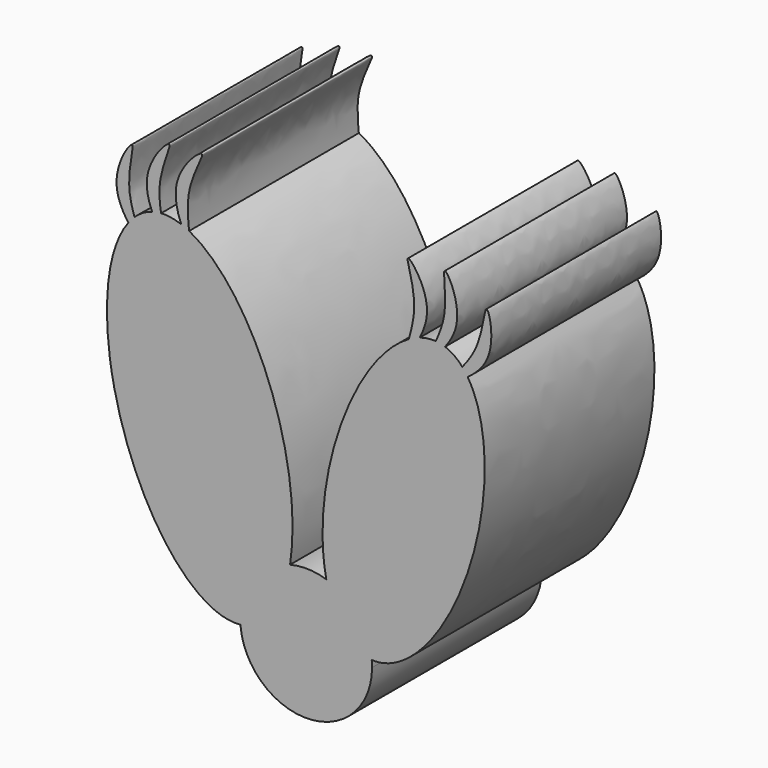
from build123d import *

# Parameters (mm, degrees)
F1_DEPTH = 25.4


# Not quite as in the source:
# - a feature of the source that left no trace in its solid (it failed there, or was rolled back) is left out


with BuildPart() as f1:
    # F0 (on Front) → F1 (new body)
    with BuildSketch(Plane.XZ):
        with BuildLine():
            ThreePointArc((-7.8657495184, -0.5963303534), (0.2983787071, -7.8826769263), (7.8883220888, 0))
            ThreePointArc((7.8883220888, 0), (7.8783514063, 0.396490223), (7.848464564, 0.7919781345))
            add(Edge.make_bspline(
                [(2.4115413859, 7.5106653182), (3.7514217892, 1.0542595546), (7.848464564, 0.7919781345)],
                knots=[2.3709530861, 2.3709530861, 2.3709530861, 3.2318966265, 3.2318966265, 3.2318966265], degree=2, weights=[1, 0.9087689813, 1]))
            ThreePointArc((2.4115413859, 7.5106653182), (0.2524493598, 7.8842814954), (-1.9261214081, 7.6495543464))
            add(Edge.make_bspline(
                [(-7.8657495184, -0.5963303534), (-3.1402244939, -0.0545859635), (-1.9261214081, 7.6495543464)],
                knots=[3.063961354, 3.063961354, 3.063961354, 3.9478311905, 3.9478311905, 3.9478311905], degree=2, weights=[1, 0.903925812, 1]))
        make_face()
        with BuildLine():
            add(Edge.make_bspline(
                [(2.4115413859, 7.5106653182), (3.7514217892, 1.0542595546), (7.848464564, 0.7919781345)],
                knots=[2.3709530861, 2.3709530861, 2.3709530861, 3.2318966265, 3.2318966265, 3.2318966265], degree=2, weights=[1, 0.9087689813, 1]))
            ThreePointArc((7.848464564, 0.7919781345), (6.1320567423, 4.9622077231), (2.4115413859, 7.5106653182))
        make_face()
        with BuildLine():
            ThreePointArc((2.4115413859, 7.5106653182), (6.1320567423, 4.9622077231), (7.848464564, 0.7919781345))
            add(Edge.make_bspline(
                [(7.848464564, 0.7919781345), (14.756882994, 0.3497201705), (19.3497784768, 13.7677159429), (23.9426739595, 27.1857117153), (19.3341341159, 34.3469906686)],
                knots=[3.2318966265, 3.2318966265, 3.2318966265, 4.5496269351, 4.5496269351, 5.8673572438, 5.8673572438, 5.8673572438], degree=2, weights=[1, 0.7906875156, 1, 0.7906875156, 1]))
            add(Edge.make_bspline(
                [(17.4727290869, 33.5254147649), (17.6220032936, 33.411960895), (18.4360560306, 33.7201138992), (19.3341341159, 34.3469906686)],
                knots=[0, 0, 0, 0, 0.1315254658, 0.1315254658, 0.1315254658, 0.1315254658], degree=3))
            add(Edge.make_bspline(
                [(18.6914906825, 35.2044384669), (17.9384272736, 34.2749423779), (17.3098526255, 33.649206847), (17.4727290869, 33.5254147649)],
                knots=[0.856489591, 0.856489591, 0.856489591, 0.856489591, 1, 1, 1, 1], degree=3))
            add(Edge.make_bspline(
                [(18.6914906825, 35.2044384669), (17.7756691464, 36.2476144498), (16.635683622, 36.651870342)],
                knots=[5.9688721424, 5.9688721424, 5.9688721424, 6.2406391942, 6.2406391942, 6.2406391942], degree=2, weights=[1, 0.9907820304, 1]))
            add(Edge.make_bspline(
                [(14.8701351136, 35.1549200714), (15.058499279, 35.0779113459), (15.8747352171, 35.6833048254), (16.635683622, 36.651870342)],
                knots=[0, 0, 0, 0, 0.1427509238, 0.1427509238, 0.1427509238, 0.1427509238], degree=3))
            add(Edge.make_bspline(
                [(15.5190667523, 36.8844184863), (15.0710606672, 35.9031366901), (14.6930112455, 35.2273334378), (14.8701351136, 35.1549200714)],
                knots=[0.8657674842, 0.8657674842, 0.8657674842, 0.8657674842, 1, 1, 1, 1], degree=3))
            add(Edge.make_bspline(
                [(15.5190667523, 36.8844184863), (14.5852576975, 36.9509876552), (13.5880398976, 36.6238878042)],
                knots=[0.0867629846, 0.0867629846, 0.0867629846, 0.2956399467, 0.2956399467, 0.2956399467], degree=2, weights=[1, 0.9945512572, 1]))
            add(Edge.make_bspline(
                [(12.1393091977, 34.898750484), (12.3347678279, 34.8563616726), (13.013036649, 35.5684327938), (13.5880398976, 36.6238878042)],
                knots=[0, 0, 0, 0, 0.14029874, 0.14029874, 0.14029874, 0.14029874], degree=3))
            add(Edge.make_bspline(
                [(12.2984461836, 36.0467759602), (12.1131626378, 35.3699550758), (11.9954319704, 34.9299529161), (12.1393091977, 34.898750484)],
                knots=[0.8967260045, 0.8967260045, 0.8967260045, 0.8967260045, 1, 1, 1, 1], degree=3))
            add(Edge.make_bspline(
                [(12.2984461836, 36.0467759602), (7.1738143092, 33.1518583115), (4.0152813166, 23.9954967618)],
                knots=[0.4297809871, 0.4297809871, 0.4297809871, 1.4031442636, 1.4031442636, 1.4031442636], degree=2, weights=[1, 0.8838897048, 1]))
            ThreePointArc((4.0152813166, 23.9954967618), (17.180368154, 14.7231281706), (2.1803673546, 8.8668232992))
            add(Edge.make_bspline(
                [(2.1803673546, 8.8668232992), (2.2756176481, 8.16563333), (2.4115413859, 7.5106653182)],
                knots=[2.2778551861, 2.2778551861, 2.2778551861, 2.3709530861, 2.3709530861, 2.3709530861], degree=2, weights=[1, 0.9989167932, 1]))
        make_face()
        with BuildLine():
            add(Edge.make_bspline(
                [(-16.8776699334, 5.1789570742), (-12.2994136592, -1.1046151815), (-7.8657495184, -0.5963303534)],
                knots=[2.2283826001, 2.2283826001, 2.2283826001, 3.063961354, 3.063961354, 3.063961354], degree=2, weights=[1, 0.9139881132, 1]))
            ThreePointArc((-7.8657495184, -0.5963303534), (-6.4006904066, 4.6105083989), (-1.9261214081, 7.6495543464))
            add(Edge.make_bspline(
                [(-1.9261214081, 7.6495543464), (1.7350735491, 30.881815249), (-14.0155701505, 38.8805496381)],
                knots=[3.9478311905, 3.9478311905, 3.9478311905, 5.8668053595, 5.8668053595, 5.8668053595], degree=2, weights=[1, 0.5739400867, 1]))
            add(Edge.make_bspline(
                [(-14.0155701505, 38.8805496381), (-13.9692331136, 38.3474513179), (-13.9585554591, 38.0149682113), (-14.0843456728, 38.01005632)],
                knots=[0.9116926893, 0.9116926893, 0.9116926893, 0.9116926893, 1, 1, 1, 1], degree=3))
            add(Edge.make_bspline(
                [(-14.0843456728, 38.01005632), (-14.2421212522, 38.0038954552), (-14.6145890314, 38.5130719057), (-14.9528763828, 39.2883132484)],
                knots=[0, 0, 0, 0, 0.1107616938, 0.1107616938, 0.1107616938, 0.1107616938], degree=3))
            add(Edge.make_bspline(
                [(-14.9528763828, 39.2883132484), (-16.2043765158, 39.7404083717), (-17.3655223204, 39.6654462324)],
                knots=[5.9522386597, 5.9522386597, 5.9522386597, 6.1810803974, 6.1810803974, 6.1810803974], degree=2, weights=[1, 0.9934610711, 1]))
            add(Edge.make_bspline(
                [(-17.3655223204, 39.6654462324), (-17.1795434662, 38.5086964495), (-16.9569761256, 37.6751636257), (-17.1571826672, 37.649743259)],
                knots=[0.8584303839, 0.8584303839, 0.8584303839, 0.8584303839, 1, 1, 1, 1], degree=3))
            add(Edge.make_bspline(
                [(-17.1571826672, 37.649743259), (-17.3543437255, 37.6247095794), (-17.9615142694, 38.3833898112), (-18.4409544135, 39.473830681)],
                knots=[0, 0, 0, 0, 0.1394161006, 0.1394161006, 0.1394161006, 0.1394161006], degree=3))
            add(Edge.make_bspline(
                [(-18.4409544135, 39.473830681), (-19.5878068307, 39.1314621905), (-20.5394386517, 38.2302190383)],
                knots=[0.0072900396, 0.0072900396, 0.0072900396, 0.2466181031, 0.2466181031, 0.2466181031], degree=2, weights=[1, 0.9928487993, 1]))
            add(Edge.make_bspline(
                [(-20.5394386517, 38.2302190383), (-20.1380049057, 37.0467661724), (-19.7331230605, 36.1979612039), (-19.9342295527, 36.1355692148)],
                knots=[0.8522933462, 0.8522933462, 0.8522933462, 0.8522933462, 1, 1, 1, 1], degree=3))
            add(Edge.make_bspline(
                [(-19.9342295527, 36.1355692148), (-20.102710459, 36.0832991028), (-20.6965090727, 36.5829791601), (-21.2904428927, 37.3886749603)],
                knots=[0, 0, 0, 0, 0.1237441449, 0.1237441449, 0.1237441449, 0.1237441449], degree=3))
            add(Edge.make_bspline(
                [(-21.2904428927, 37.3886749603), (-25.6133300033, 31.7080986333), (-22.9671125849, 19.4320361213)],
                knots=[0.3465956992, 0.3465956992, 0.3465956992, 1.4408599981, 1.4408599981, 1.4408599981], degree=2, weights=[1, 0.854020003, 1]))
            ThreePointArc((-22.9671125849, 19.4320361213), (-7.0630025292, 17.7995031872), (-16.8776699334, 5.1789570742))
        make_face()
        with BuildLine():
            ThreePointArc((-1.9261214081, 7.6495543464), (-6.4006904066, 4.6105083989), (-7.8657495184, -0.5963303534))
            add(Edge.make_bspline(
                [(-7.8657495184, -0.5963303534), (-3.1402244939, -0.0545859635), (-1.9261214081, 7.6495543464)],
                knots=[3.063961354, 3.063961354, 3.063961354, 3.9478311905, 3.9478311905, 3.9478311905], degree=2, weights=[1, 0.903925812, 1]))
        make_face()
        with BuildLine():
            add(Edge.make_bspline(
                [(17.4727290869, 33.5254147649), (17.6220032936, 33.411960895), (18.4360560306, 33.7201138992), (19.3341341159, 34.3469906686)],
                knots=[0, 0, 0, 0, 0.1315254658, 0.1315254658, 0.1315254658, 0.1315254658], degree=3))
            add(Edge.make_bspline(
                [(19.3341341159, 34.3469906686), (19.0317675739, 34.8168425581), (18.6914906825, 35.2044384669)],
                knots=[5.8673572438, 5.8673572438, 5.8673572438, 5.9688721424, 5.9688721424, 5.9688721424], degree=2, weights=[1, 0.9987121172, 1]))
            add(Edge.make_bspline(
                [(18.6914906825, 35.2044384669), (17.9384272736, 34.2749423779), (17.3098526255, 33.649206847), (17.4727290869, 33.5254147649)],
                knots=[0.856489591, 0.856489591, 0.856489591, 0.856489591, 1, 1, 1, 1], degree=3))
        make_face()
        with BuildLine():
            add(Edge.make_bspline(
                [(19.3341341159, 34.3469906686), (19.0317675739, 34.8168425581), (18.6914906825, 35.2044384669)],
                knots=[5.8673572438, 5.8673572438, 5.8673572438, 5.9688721424, 5.9688721424, 5.9688721424], degree=2, weights=[1, 0.9987121172, 1]))
            add(Edge.make_bspline(
                [(19.3341341159, 34.3469906686), (20.1798236278, 34.9372991482), (23.0009000721, 37.6134714521), (21.297221073, 45.0520380481), (21.2424649704, 38.6066952932), (19.2203684111, 35.8572251704), (18.6914906825, 35.2044384669)],
                knots=[0.1315254658, 0.1315254658, 0.1315254658, 0.1315254658, 0.2553785124, 0.5112252974, 0.7557019837, 0.856489591, 0.856489591, 0.856489591, 0.856489591], degree=3))
        make_face()
        with BuildLine():
            add(Edge.make_bspline(
                [(-22.9671125849, 19.4320361213), (-21.1623610737, 11.0596166006), (-16.8776699334, 5.1789570742)],
                knots=[1.4408599981, 1.4408599981, 1.4408599981, 2.2283826001, 2.2283826001, 2.2283826001], degree=2, weights=[1, 0.9234725177, 1]))
            ThreePointArc((-16.8776699334, 5.1789570742), (-7.0630025292, 17.7995031872), (-22.9671125849, 19.4320361213))
        make_face()
        with BuildLine():
            add(Edge.make_bspline(
                [(4.0152813166, 23.9954967618), (1.2243313225, 15.9047320704), (2.1803673546, 8.8668232992)],
                knots=[1.4031442636, 1.4031442636, 1.4031442636, 2.2778551861, 2.2778551861, 2.2778551861], degree=2, weights=[1, 0.9058749116, 1]))
            ThreePointArc((2.1803673546, 8.8668232992), (17.180368154, 14.7231281706), (4.0152813166, 23.9954967618))
        make_face()
        with BuildLine():
            add(Edge.make_bspline(
                [(-14.0155701505, 38.8805496381), (-13.9692331136, 38.3474513179), (-13.9585554591, 38.0149682113), (-14.0843456728, 38.01005632)],
                knots=[0.9116926893, 0.9116926893, 0.9116926893, 0.9116926893, 1, 1, 1, 1], degree=3))
            add(Edge.make_bspline(
                [(-14.0155701505, 38.8805496381), (-14.4874124644, 39.1201678667), (-14.9528763828, 39.2883132484)],
                knots=[5.8668053595, 5.8668053595, 5.8668053595, 5.9522386597, 5.9522386597, 5.9522386597], degree=2, weights=[1, 0.9990877826, 1]))
            add(Edge.make_bspline(
                [(-14.0843456728, 38.01005632), (-14.2421212522, 38.0038954552), (-14.6145890314, 38.5130719057), (-14.9528763828, 39.2883132484)],
                knots=[0, 0, 0, 0, 0.1107616938, 0.1107616938, 0.1107616938, 0.1107616938], degree=3))
        make_face()
        with BuildLine():
            add(Edge.make_bspline(
                [(-14.0155701505, 38.8805496381), (-14.4874124644, 39.1201678667), (-14.9528763828, 39.2883132484)],
                knots=[5.8668053595, 5.8668053595, 5.8668053595, 5.9522386597, 5.9522386597, 5.9522386597], degree=2, weights=[1, 0.9990877826, 1]))
            add(Edge.make_bspline(
                [(-14.9528763828, 39.2883132484), (-15.3945637468, 40.3005127993), (-16.4563018581, 44.3594325367), (-10.6057865956, 49.6457518305), (-14.5932155129, 43.8468818401), (-14.0974223439, 39.8222427148), (-14.0155701505, 38.8805496381)],
                knots=[0.1107616938, 0.1107616938, 0.1107616938, 0.1107616938, 0.2553785124, 0.5112252974, 0.7557019837, 0.9116926893, 0.9116926893, 0.9116926893, 0.9116926893], degree=3))
        make_face()
        with BuildLine():
            add(Edge.make_bspline(
                [(14.8701351136, 35.1549200714), (15.058499279, 35.0779113459), (15.8747352171, 35.6833048254), (16.635683622, 36.651870342)],
                knots=[0, 0, 0, 0, 0.1427509238, 0.1427509238, 0.1427509238, 0.1427509238], degree=3))
            add(Edge.make_bspline(
                [(16.635683622, 36.651870342), (16.4582878028, 36.7147775488), (16.2765569985, 36.7615083232)],
                knots=[6.2406391942, 6.2406391942, 6.2406391942, 6.2831853072, 6.2831853072, 6.2831853072], degree=2, weights=[1, 0.9997737371, 1]))
            add(Edge.make_bspline(
                [(16.2765569985, 36.7615083232), (15.9057822203, 36.8568504014), (15.5190667523, 36.8844184863)],
                knots=[0, 0, 0, 0.0867629846, 0.0867629846, 0.0867629846], degree=2, weights=[1, 0.9990591706, 1]))
            add(Edge.make_bspline(
                [(15.5190667523, 36.8844184863), (15.0710606672, 35.9031366901), (14.6930112455, 35.2273334378), (14.8701351136, 35.1549200714)],
                knots=[0.8657674842, 0.8657674842, 0.8657674842, 0.8657674842, 1, 1, 1, 1], degree=3))
        make_face()
        with BuildLine():
            add(Edge.make_bspline(
                [(16.635683622, 36.651870342), (16.4582878028, 36.7147775488), (16.2765569985, 36.7615083232)],
                knots=[6.2406391942, 6.2406391942, 6.2406391942, 6.2831853072, 6.2831853072, 6.2831853072], degree=2, weights=[1, 0.9997737371, 1]))
            add(Edge.make_bspline(
                [(16.635683622, 36.651870342), (17.2360565062, 37.4160489236), (19.0876512511, 40.6557653869), (15.581001064, 47.2786345544), (17.2212194556, 40.9424294881), (15.8864145121, 37.6890318199), (15.5190667523, 36.8844184863)],
                knots=[0.1427509238, 0.1427509238, 0.1427509238, 0.1427509238, 0.2553785124, 0.5112252974, 0.7557019837, 0.8657674842, 0.8657674842, 0.8657674842, 0.8657674842], degree=3))
            add(Edge.make_bspline(
                [(16.2765569985, 36.7615083232), (15.9057822203, 36.8568504014), (15.5190667523, 36.8844184863)],
                knots=[0, 0, 0, 0.0867629846, 0.0867629846, 0.0867629846], degree=2, weights=[1, 0.9990591706, 1]))
        make_face()
        with BuildLine():
            add(Edge.make_bspline(
                [(-21.2904428927, 37.3886749603), (-21.9222473541, 38.2457438523), (-23.7824880294, 41.7879552231), (-19.585739103, 48.2751053539), (-21.7236926746, 42.2421476598), (-20.8019524346, 39.0041267923), (-20.5394386517, 38.2302190383)],
                knots=[0.1237441449, 0.1237441449, 0.1237441449, 0.1237441449, 0.2553785124, 0.5112252974, 0.7557019837, 0.8522933462, 0.8522933462, 0.8522933462, 0.8522933462], degree=3))
            add(Edge.make_bspline(
                [(-20.5394386517, 38.2302190383), (-20.9354066326, 37.8552174637), (-21.2904428927, 37.3886749603)],
                knots=[0.2466181031, 0.2466181031, 0.2466181031, 0.3465956992, 0.3465956992, 0.3465956992], degree=2, weights=[1, 0.9987508202, 1]))
        make_face()
        with BuildLine():
            add(Edge.make_bspline(
                [(-20.5394386517, 38.2302190383), (-20.9354066326, 37.8552174637), (-21.2904428927, 37.3886749603)],
                knots=[0.2466181031, 0.2466181031, 0.2466181031, 0.3465956992, 0.3465956992, 0.3465956992], degree=2, weights=[1, 0.9987508202, 1]))
            add(Edge.make_bspline(
                [(-19.9342295527, 36.1355692148), (-20.102710459, 36.0832991028), (-20.6965090727, 36.5829791601), (-21.2904428927, 37.3886749603)],
                knots=[0, 0, 0, 0, 0.1237441449, 0.1237441449, 0.1237441449, 0.1237441449], degree=3))
            add(Edge.make_bspline(
                [(-20.5394386517, 38.2302190383), (-20.1380049057, 37.0467661724), (-19.7331230605, 36.1979612039), (-19.9342295527, 36.1355692148)],
                knots=[0.8522933462, 0.8522933462, 0.8522933462, 0.8522933462, 1, 1, 1, 1], degree=3))
        make_face()
        with BuildLine():
            add(Edge.make_bspline(
                [(13.5880398976, 36.6238878042), (14.0596852095, 37.4896227521), (15.3559565763, 41.0247326105), (10.7341145705, 46.9617190791), (13.5874167288, 40.7045562879), (12.5514569295, 36.9709970293), (12.2984461836, 36.0467759602)],
                knots=[0.14029874, 0.14029874, 0.14029874, 0.14029874, 0.2553785124, 0.5112252974, 0.7557019837, 0.8967260045, 0.8967260045, 0.8967260045, 0.8967260045], degree=3))
            add(Edge.make_bspline(
                [(13.5880398976, 36.6238878042), (12.9489969981, 36.4142737787), (12.2984461836, 36.0467759602)],
                knots=[0.2956399467, 0.2956399467, 0.2956399467, 0.4297809871, 0.4297809871, 0.4297809871], degree=2, weights=[1, 0.9977516157, 1]))
        make_face()
        with BuildLine():
            add(Edge.make_bspline(
                [(13.5880398976, 36.6238878042), (12.9489969981, 36.4142737787), (12.2984461836, 36.0467759602)],
                knots=[0.2956399467, 0.2956399467, 0.2956399467, 0.4297809871, 0.4297809871, 0.4297809871], degree=2, weights=[1, 0.9977516157, 1]))
            add(Edge.make_bspline(
                [(12.2984461836, 36.0467759602), (12.1131626378, 35.3699550758), (11.9954319704, 34.9299529161), (12.1393091977, 34.898750484)],
                knots=[0.8967260045, 0.8967260045, 0.8967260045, 0.8967260045, 1, 1, 1, 1], degree=3))
            add(Edge.make_bspline(
                [(12.1393091977, 34.898750484), (12.3347678279, 34.8563616726), (13.013036649, 35.5684327938), (13.5880398976, 36.6238878042)],
                knots=[0, 0, 0, 0, 0.14029874, 0.14029874, 0.14029874, 0.14029874], degree=3))
        make_face()
        with BuildLine():
            add(Edge.make_bspline(
                [(-17.3655223204, 39.6654462324), (-17.1795434662, 38.5086964495), (-16.9569761256, 37.6751636257), (-17.1571826672, 37.649743259)],
                knots=[0.8584303839, 0.8584303839, 0.8584303839, 0.8584303839, 1, 1, 1, 1], degree=3))
            add(Edge.make_bspline(
                [(-17.3655223204, 39.6654462324), (-17.8817895896, 39.632116655), (-18.3712700382, 39.4940581173)],
                knots=[6.1810803974, 6.1810803974, 6.1810803974, 6.2831853072, 6.2831853072, 6.2831853072], degree=2, weights=[1, 0.9986971064, 1]))
            add(Edge.make_bspline(
                [(-18.3712700382, 39.4940581173), (-18.4061875265, 39.4842095985), (-18.4409544135, 39.473830681)],
                knots=[0, 0, 0, 0.0072900396, 0.0072900396, 0.0072900396], degree=2, weights=[1, 0.9999933569, 1]))
            add(Edge.make_bspline(
                [(-17.1571826672, 37.649743259), (-17.3543437255, 37.6247095794), (-17.9615142694, 38.3833898112), (-18.4409544135, 39.473830681)],
                knots=[0, 0, 0, 0, 0.1394161006, 0.1394161006, 0.1394161006, 0.1394161006], degree=3))
        make_face()
        with BuildLine():
            add(Edge.make_bspline(
                [(-17.3655223204, 39.6654462324), (-17.8817895896, 39.632116655), (-18.3712700382, 39.4940581173)],
                knots=[6.1810803974, 6.1810803974, 6.1810803974, 6.2831853072, 6.2831853072, 6.2831853072], degree=2, weights=[1, 0.9986971064, 1]))
            add(Edge.make_bspline(
                [(-18.4409544135, 39.473830681), (-18.8397393117, 40.3808288882), (-19.835020981, 44.0248585135), (-14.7059782421, 49.5443378352), (-17.8914813012, 43.9170189047), (-17.5004757849, 40.504828707), (-17.3655223204, 39.6654462324)],
                knots=[0.1394161006, 0.1394161006, 0.1394161006, 0.1394161006, 0.2553785124, 0.5112252974, 0.7557019837, 0.8584303839, 0.8584303839, 0.8584303839, 0.8584303839], degree=3))
            add(Edge.make_bspline(
                [(-18.3712700382, 39.4940581173), (-18.4061875265, 39.4842095985), (-18.4409544135, 39.473830681)],
                knots=[0, 0, 0, 0.0072900396, 0.0072900396, 0.0072900396], degree=2, weights=[1, 0.9999933569, 1]))
        make_face()
    extrude(amount=F1_DEPTH)


solid = f1.part
